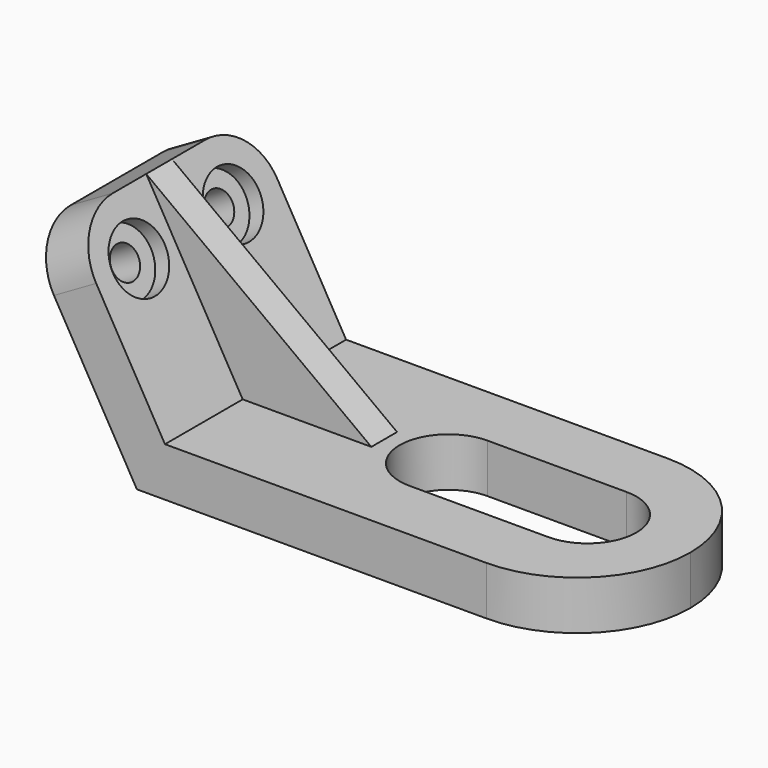
from build123d import *

# Parameters (mm, degrees)
F1_DEPTH = 22.352
F2_DEPTH = 3.175
F4_R     = 22.35199
F5_DEPTH = 25.4
F6_R     = 3.175
F7_DEPTH = 25.4
F8_R     = 6.35
F8_R_2   = 3.175
F9_DEPTH = 3.175
F10_R    = 10.922


# Not quite as in the source:
# - a fillet or chamfer is up to 0.001 mm smaller than in the source, because OpenCascade refuses the exact size


with BuildPart() as f1:
    # F0 (on Front) → F1 (new body, symmetric)
    with BuildSketch(Plane.XZ):
        Polygon((0, 0), (-25.4, 0), (-44.45, 32.9955678842), (-52.7857543947, 28.1829178405), (-30.9417543947, -9.652), (60.452, -9.652), (60.452, 0), align=None)
    extrude(amount=F1_DEPTH, both=True)

    # F0 (on Front) → F2 (join, symmetric)
    with BuildSketch(Plane.XZ):
        Polygon((-44.45, 32.9955678842), (-25.4, 0), (0, 0), align=None)
    extrude(amount=F2_DEPTH, both=True)

    # F4 (radius 22.352 in the source; OpenCascade refuses exactly that, so slightly less here)
    f4_edges = [f1.edges().sort_by_distance(p)[0] for p in [
        (60.452, -22.352, -4.826),
        (60.452, 22.352, -4.826),
    ]]
    fillet(f4_edges, radius=F4_R)

    # F3 (on face) → F5 (cut)
    with BuildSketch(Plane.XY):
        with BuildLine():
            ThreePointArc((12.7, 9.652), (3.048, 0), (12.7, -9.652))
            Line((12.7, -9.652), (40.1388603866, -9.652))
            ThreePointArc((40.1388603866, -9.652), (49.7908603866, 0), (40.1388603866, 9.652))
            Line((40.1388603866, 9.652), (12.7, 9.652))
        make_face()
    extrude(amount=-F5_DEPTH, mode=Mode.SUBTRACT)

    # F6 (on face) → F7 (cut)
    with BuildSketch(Plane(origin=(-27.3857543947, 0, -15.8111726717), x_dir=(0, -1, 0), z_dir=(-0.8660254038, 0, -0.5))):
        with Locations((11.8134439608, 39.878)):
            Circle(F6_R)
        with Locations((-11.43, 39.878)):
            Circle(F6_R)
    extrude(amount=-F7_DEPTH, mode=Mode.SUBTRACT)

    # F8 (on face) → F9 (cut)
    with BuildSketch(Plane(origin=(-19.05, 0, -10.9985226281), x_dir=(0, 1, 0), z_dir=(0.8660254038, 0, 0.5))):
        with Locations((-11.8134439608, 39.878)):
            Circle(F8_R)
        with Locations((-11.8134439608, 39.878)):
            Circle(F8_R_2, mode=Mode.SUBTRACT)
        with Locations((11.43, 39.878)):
            Circle(F8_R)
    extrude(amount=-F9_DEPTH, mode=Mode.SUBTRACT)

    # F10
    f10_edges = [f1.edges().sort_by_distance(p)[0] for p in [
        (-48.617877, -22.352, 30.589243),
        (-48.617877, 22.352, 30.589243),
    ]]
    fillet(f10_edges, radius=F10_R)


solid = f1.part
